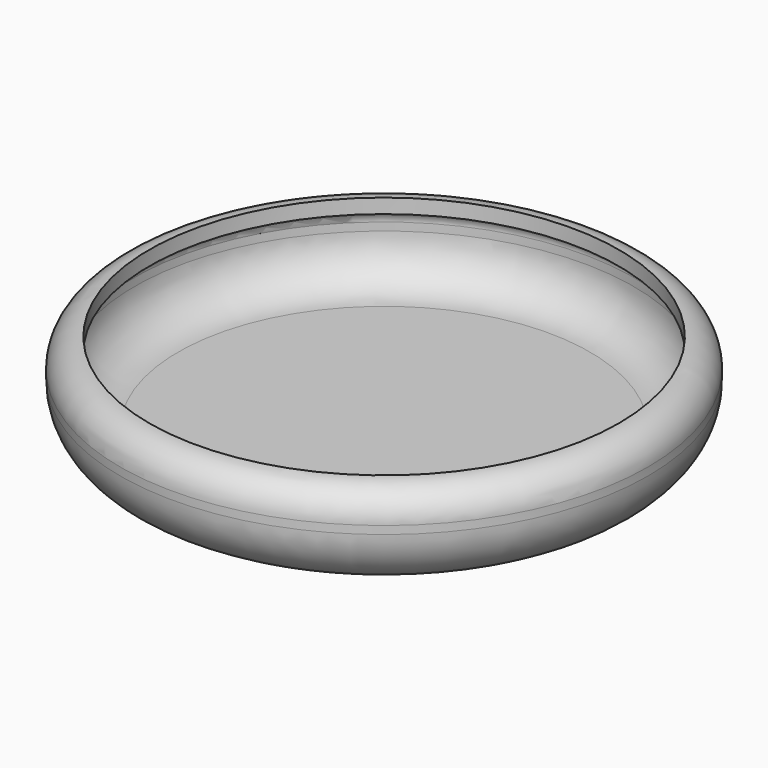
from build123d import *

# Parameters (mm, degrees)
F0_R     = 18.1702284577
F1_DEPTH = 6.5465988591
F2_R     = 4
F3_R     = 2
F4_T     = -1


# Not quite as in the source:
# - a shell that OpenCascade refuses in one call is made with other operations: the cavity is built on its own and cut out


with BuildPart() as f1:
    # F0 (on Top) → F1 (new body)
    with BuildSketch(Plane.XY):
        Circle(F0_R)
    extrude(amount=F1_DEPTH)

    # F2
    f2_edges = [f1.edges().sort_by_distance(p)[0] for p in [
        (-18.170228, 0, 0),
    ]]
    fillet(f2_edges, radius=F2_R)

    # F3
    f3_edges = [f1.edges().sort_by_distance(p)[0] for p in [
        (-18.170228, 0, 6.546599),
    ]]
    fillet(f3_edges, radius=F3_R)

    # F4: a shell. OpenCascade refuses it in one call, so the cavity is built on its own and cut out:
    # the body offset inwards by the wall thickness, plus a prism from it out through each open face.
    f4_core = offset(f1.part, amount=F4_T, mode=Mode.PRIVATE)
    f4_exits = [f4_core.faces().sort_by_distance(p)[0] for p in [
        (0, 0, 5.546599),
    ]]
    add(f4_core, mode=Mode.SUBTRACT)
    extrude(f4_exits, amount=-F4_T, mode=Mode.SUBTRACT)


solid = f1.part
